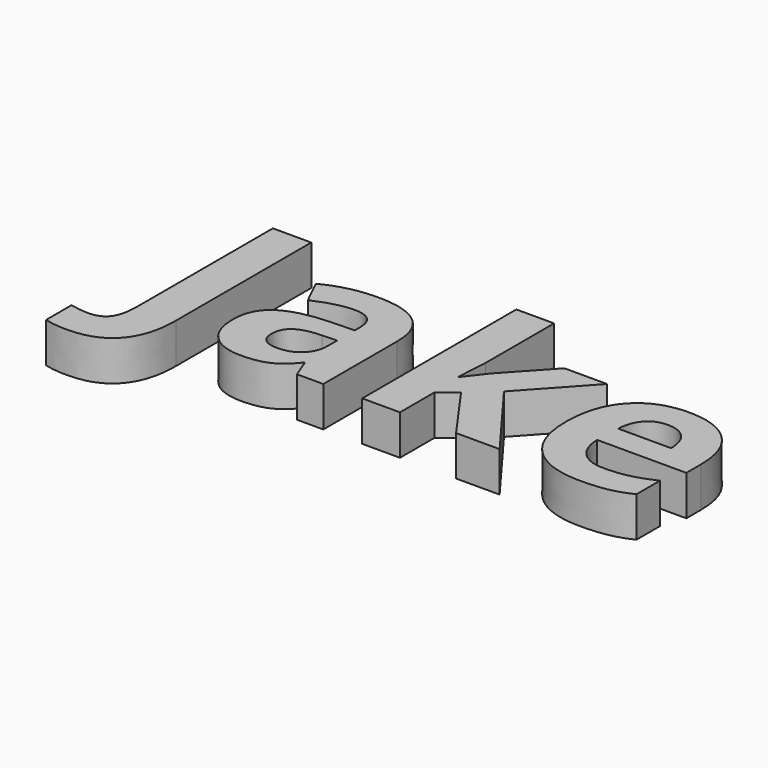
from build123d import *

# Parameters (mm, degrees)
F0_TEXT_SIZE = 40.2166676294
F1_DEPTH     = 6.35


# Not quite as in the source:
# - Text() gives the source's letters only with a copy of the font that has no kerning and outlines rounded to 1/6400 em; it was checked with that copy


with BuildPart() as f1:
    # F0 (on Top) → F1 (new body)
    with BuildSketch(Plane.XY):
        with Locations((-30.1751997322, -19.0500002354)):
            Text('Jake', F0_TEXT_SIZE, font='Open Sans', font_style=FontStyle.BOLD, text_align=(TextAlign.LEFT, TextAlign.BOTTOM))
    extrude(amount=F1_DEPTH)


solid = f1.part
